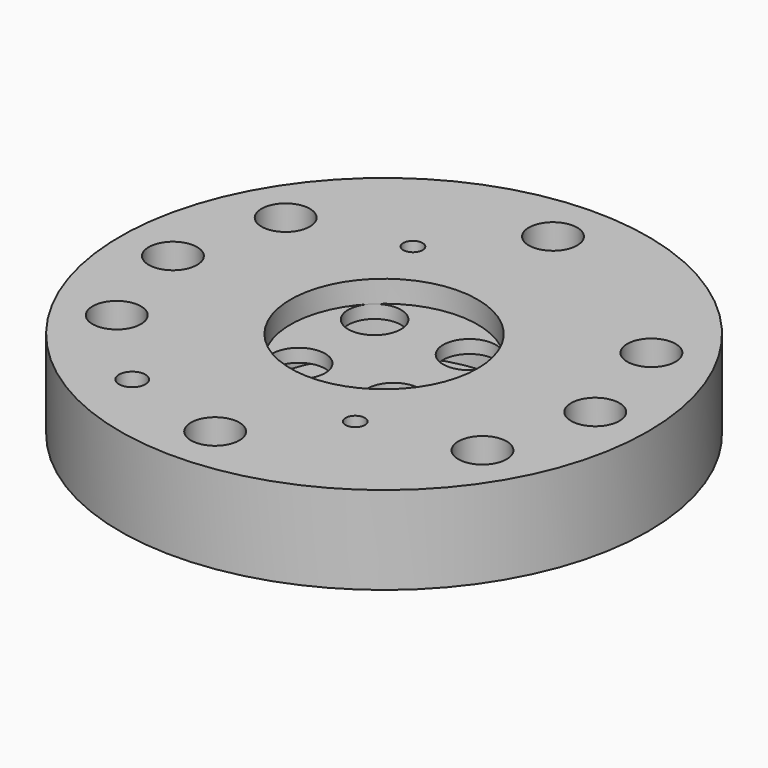
from build123d import *

# Parameters (mm, degrees)
F0_R            = 60
F1_DEPTH        = 20
F2_R            = 21.25
F3_DEPTH        = 5
F4_R            = 6
F5_DEPTH        = 20.001
F6_R            = 30
F7_DEPTH        = 12
F8_R            = 8.5
F9_DEPTH        = 11
F10_R           = 5.5
F11_DEPTH       = 9.001
F12_R           = 5.5
F13_DEPTH       = 20.001
F15_D           = 4.4
F16_R           = 38
F17_DEPTH       = 5
F19_D           = 4.4
F19_CSINK_D     = 8.96
F19_CSINK_ANGLE = 90
F20_T2_ANGLE    = 181.12451927
F20_T4_ANGLE    = 120.559173381
F20_T6_ANGLE    = 60.5572258986
F22_D           = 10.3
F22_DEPTH       = 20.25
F22_TIP         = 3.094432188
F23_R           = 3
F24_DEPTH       = 25
F26_DEPTH       = 7


# Not quite as in the source:
# - a fillet or chamfer that OpenCascade refuses, or shapes differently, is made with other operations: its cross-section is extruded or revolved along the edge and cut away or added
# - a pattern or mirror of a feature is missing from the dataset's text; its kind, count and spacing are read off the source's solid


with BuildPart() as f1:
    # F0 (on Top) → F1 (new body)
    with BuildSketch(Plane.XY):
        Circle(F0_R)
    extrude(amount=F1_DEPTH)

    # F2 (on face) → F3 (cut)
    with BuildSketch(Plane.XY.offset(20)):
        Circle(F2_R)
    extrude(amount=-F3_DEPTH, mode=Mode.SUBTRACT)

    # F4 (on face) → F5 (cut, through all)
    with BuildSketch(Plane.XY.offset(20)):
        with Locations((10.7833784131, 10.7833784131)):
            Circle(F4_R)
        with Locations((-10.7833784131, 10.7833784131)):
            Circle(F4_R)
        with Locations((-10.7833784131, -10.7833784131)):
            Circle(F4_R)
        with Locations((10.7833784131, -10.7833784131)):
            Circle(F4_R)
    extrude(amount=-F5_DEPTH, mode=Mode.SUBTRACT)

    # F6 (on face) → F7 (cut)
    with BuildSketch(Plane(origin=(0, 0, 0), x_dir=(1, 0, 0), z_dir=(0, 0, -1))):
        Circle(F6_R)
    extrude(amount=-F7_DEPTH, mode=Mode.SUBTRACT)

    # F8 (on face) → F9 (cut)
    with BuildSketch(Plane(origin=(0, 0, 0), x_dir=(1, 0, 0), z_dir=(0, 0, -1))):
        with Locations((-48, 0)):
            Circle(F8_R)
        with Locations((48, 0)):
            Circle(F8_R)
    extrude(amount=-F9_DEPTH, mode=Mode.SUBTRACT)

    # F10 (on face) → F11 (cut, through all)
    with BuildSketch(Plane(origin=(0, 0, 11), x_dir=(1, 0, 0), z_dir=(0, 0, -1))):
        with Locations((-48, 0)):
            Circle(F10_R)
        with Locations((48, 0)):
            Circle(F10_R)
    extrude(amount=-F11_DEPTH, mode=Mode.SUBTRACT)

    # F12 (on face) → F13 (cut, through all)
    with BuildSketch(Plane(origin=(0, 0, 0), x_dir=(1, 0, 0), z_dir=(0, 0, -1))):
        with Locations((41.5692193817, 24)):
            Circle(F12_R)
        with Locations((0, 48)):
            Circle(F12_R)
        with Locations((-41.5692193817, 24)):
            Circle(F12_R)
        with Locations((-41.5692193817, -24)):
            Circle(F12_R)
        with Locations((0, -48)):
            Circle(F12_R)
        with Locations((41.5692193817, -24)):
            Circle(F12_R)
    extrude(amount=-F13_DEPTH, mode=Mode.SUBTRACT)

    # F15 (through all)
    with Locations(Plane(origin=(0, 0, 0), x_dir=(1, 0, 0), z_dir=(0, 0, -1))):
        with Locations((17, 29.4448637287)):
            f15 = Hole(F15_D / 2)

    # F15_copies: F15 across plane
    add(f15.mirror(Plane(origin=(0, 0, 0), x_dir=(0.8660254038, 0.5, 0), z_dir=(-0.5, 0.8660254038, 0))), mode=Mode.SUBTRACT)

    # F23 (on face) → F24 (cut)
    with BuildSketch(Plane(origin=(0, 0, 0), x_dir=(1, 0, 0), z_dir=(0, 0, -1))):
        with Locations((-24, 41.5692193817)):
            Circle(F23_R)
    extrude(amount=-F24_DEPTH, mode=Mode.SUBTRACT)

    # F25 (on face) → F26 (cut)
    with BuildSketch(Plane(origin=(0, 0, 0), x_dir=(1, 0, 0), z_dir=(0, 0, -1))):
        with BuildLine():
            ThreePointArc((-21.8349364905, 42.8192193817), (-25.25, 43.7342828911), (-26.1650635095, 40.3192193817))
            Line((-26.1650635095, 40.3192193817), (-17.1128894383, 24.6403939715))
            ThreePointArc((-17.1128894383, 24.6403939715), (-16.0704251253, 25.332616057), (-15, 25.9807621135))
            ThreePointArc((-15, 25.9807621135), (-13.903476487, 26.5837044366), (-12.7827624194, 27.1403939715))
            Line((-12.7827624194, 27.1403939715), (-21.8349364905, 42.8192193817))
        make_face()
    extrude(amount=-F26_DEPTH, mode=Mode.SUBTRACT)


with BuildPart() as f17:
    # F16 (on face) → F17 (new body)
    with BuildSketch(Plane(origin=(0, 0, 0), x_dir=(1, 0, 0), z_dir=(0, 0, -1))):
        Circle(F16_R)
    extrude(amount=F17_DEPTH)

    # F19 (through all)
    with Locations(Plane(origin=(0, 0, -5), x_dir=(1, 0, 0), z_dir=(0, 0, -1))):
        with Locations((17, 29.4448637287)):
            f19 = CounterSinkHole(F19_D / 2, F19_CSINK_D / 2, counter_sink_angle=F19_CSINK_ANGLE)

    # F19_copies: F19 across plane
    add(f19.mirror(Plane(origin=(0, 0, 0), x_dir=(0.8660254038, 0.5, 0), z_dir=(-0.5, 0.8660254038, 0))), mode=Mode.SUBTRACT)

    # F20: fillet of radius 1 on 3 edges, made by hand

    # F20_s1 → F20_t2 (revolve, cut)
    with BuildSketch(Plane(origin=(0, 0, 0), x_dir=(0, 0, 1), z_dir=(0.8610771426, 0.5084743401, 0))):
        with BuildLine():
            ThreePointArc((-4, 38), (-4.7071067812, 37.7071067812), (-5, 37))
            Line((-5, 37), (-5, 38))
            Line((-5, 38), (-4, 38))
        make_face()
    revolve(axis=Axis((0, 0, -5), (0, 0, -1)), revolution_arc=F20_T2_ANGLE, mode=Mode.SUBTRACT)

    # F20_s3 → F20_t4 (revolve, cut)
    with BuildSketch(Plane(origin=(0, 0, 0), x_dir=(0, 0, 1), z_dir=(-0.8611045305, -0.5084279572, 0))):
        with BuildLine():
            ThreePointArc((-4, 38), (-4.7071067812, 37.7071067812), (-5, 37))
            Line((-5, 37), (-5, 38))
            Line((-5, 38), (-4, 38))
        make_face()
    revolve(axis=Axis((0, 0, -5), (0, 0, -1)), revolution_arc=F20_T4_ANGLE, mode=Mode.SUBTRACT)

    # F20_s5 → F20_t6 (revolve, cut)
    with BuildSketch(Plane.XZ):
        with BuildLine():
            ThreePointArc((38, -4), (37.7071067812, -4.7071067812), (37, -5))
            Line((37, -5), (38, -5))
            Line((38, -5), (38, -4))
        make_face()
    revolve(axis=Axis((0, 0, -5), (0, 0, -1)), revolution_arc=F20_T6_ANGLE, mode=Mode.SUBTRACT)

    # F22
    with Locations(Plane(origin=(0, 0, -5), x_dir=(1, 0, 0), z_dir=(0, 0, -1))):
        with Locations((0, 0)):
            Hole(F22_D / 2, depth=F22_DEPTH)
            with Locations((0, 0, -(F22_DEPTH + F22_TIP / 2))):  # 118° drill point
                Cone(0, F22_D / 2, F22_TIP, mode=Mode.SUBTRACT)


solid = Compound([f1.part, f17.part])
